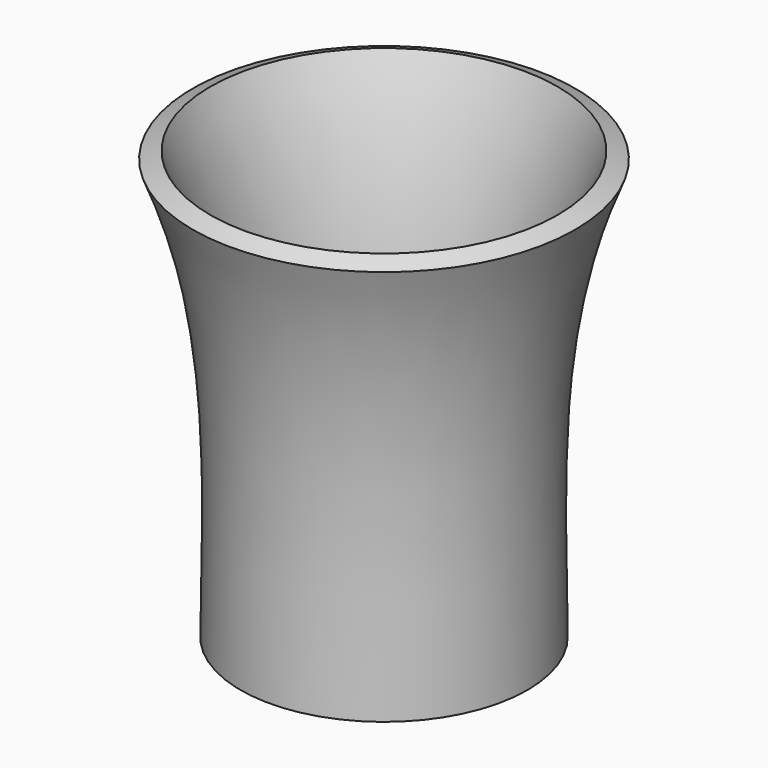
from build123d import *


with BuildPart() as f1:
    # F0 (on Front) → F1 (revolve)
    with BuildSketch(Plane.XZ):
        with BuildLine():
            add(Edge.make_bspline(
                [(19.7018157983, 0), (19.2818126331, 25.5410025517), (18.5987663766, 46.3006769617), (27.4861888909, 67.7786726008)],
                knots=[0, 0, 0, 0, 68.2242253453, 68.2242253453, 68.2242253453, 68.2242253453], degree=3))
            Line((19.7018157983, 0), (22.7014102595, 0.0493261439))
            add(Edge.make_bspline(
                [(22.7014102595, 0.0493261439), (22.5962995232, 6.4412626981), (22.3545888627, 18.5799406922), (22.8112736431, 35.3311021878), (24.9650033553, 51.1343432532), (28.1068589741, 61.4324338738), (30.2582404805, 66.6316198626)],
                knots=[0, 0, 0, 0, 0.25, 0.5, 0.75, 1, 1, 1, 1], degree=3))
            Line((30.2582404805, 66.6316198626), (27.4861888909, 67.7786726008))
        make_face()
    revolve(axis=Axis((0, 0, 30.712608248), (0, 0, 1)))


solid = f1.part
